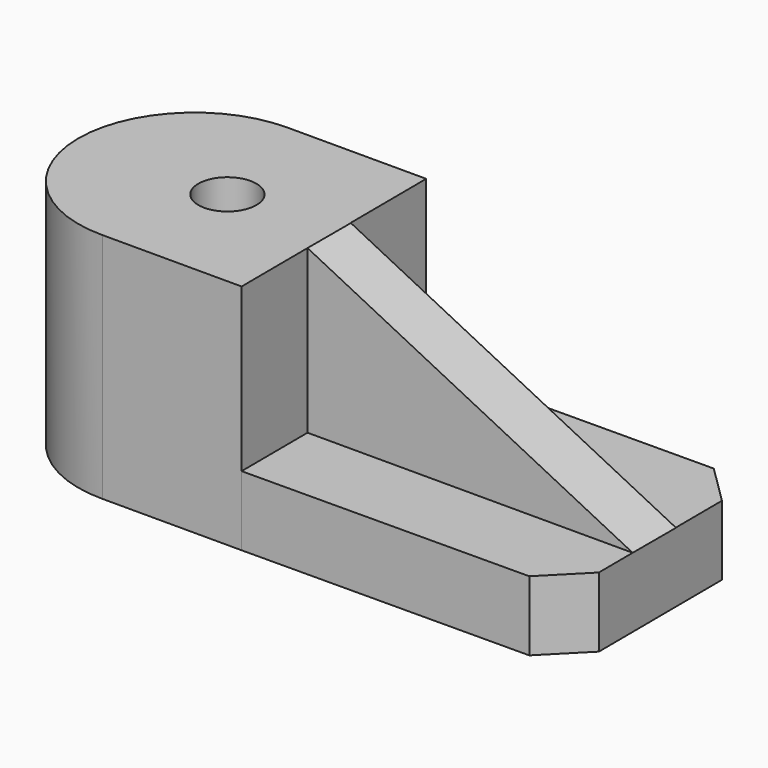
from build123d import *

# Parameters (mm, degrees)
F1_DEPTH  = 30
F2_R      = 3.75
F3_DEPTH  = 30
F4_W      = 30.0004304858
F4_H      = 9
F5_DEPTH  = 42
F6_SIZE   = 5
F7_W      = 0.0346347876
F7_H      = 6.4651286568
F8_DEPTH  = 21
F10_DEPTH = 25


with BuildPart() as f1:
    # F0 (on Top) → F1 (new body)
    with BuildSketch(Plane.XY):
        with BuildLine():
            Line((8.7358052025, -10.7137067538), (8.5750901289, 19.2862932462))
            Line((8.5750901289, 19.2862932462), (-9.4249098711, 19.2862932462))
            ThreePointArc((-9.4249098711, 19.2862932462), (-24.3445523343, 4.2059357094), (-9.2641947975, -10.7137067538))
            Line((-9.2641947975, -10.7137067538), (8.7358052025, -10.7137067538))
        make_face()
    extrude(amount=F1_DEPTH)

    # F2 (on face) → F3 (cut)
    with BuildSketch(Plane.XY.offset(30)):
        with Locations((-4.9572857097, 4.1074641049)):
            Circle(F2_R)
    extrude(amount=-F3_DEPTH, mode=Mode.SUBTRACT)

    # F4 (on face) → F5 (join)
    with BuildSketch(Plane(origin=(8.6781610067, 0.0464903762, 0), x_dir=(-0.0053570922, 0.9999856507, 0), z_dir=(0.9999856507, 0.0053570922, 0))):
        with Locations((4.2398637092, 4.5)):
            Rectangle(F4_W, F4_H)
    extrude(amount=F5_DEPTH)

    # F6
    f6_edges = [f1.edges().sort_by_distance(p)[0] for p in [
        (50.735203, -10.488709, 4.5),
        (50.574487, 19.511291, 4.5),
    ]]
    chamfer(f6_edges, length=F6_SIZE)

    # F7 (on face) → F8 (join)
    with BuildSketch(Plane.XY.offset(9)):
        with Locations((50.6616953499, 3.2325643284)):
            Rectangle(F7_W, F7_H)
        Polygon((8.6409098797, 0), (50.6443779561, 0), (50.6443779561, 6.4651286568), (50.6790127437, 6.4651286568), (50.6790127437, 7), (8.6409098797, 7), align=None)
    extrude(amount=F8_DEPTH)

    # F9 (on face) → F10 (cut)
    with BuildSketch(Plane.XZ):
        Polygon((50.6790127437, 30), (8.6784100635, 30), (50.6790127437, 9), align=None)
    extrude(amount=-F10_DEPTH, mode=Mode.SUBTRACT)


solid = f1.part
